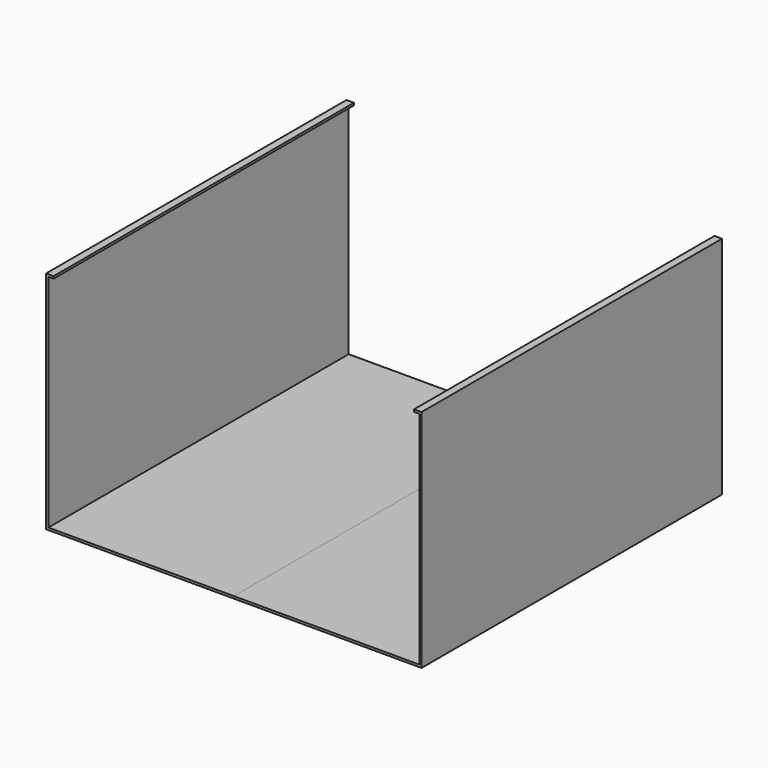
from build123d import *

# Parameters (mm, degrees)
F1_DEPTH = 6350


# Not quite as in the source:
# - a pattern or mirror of a feature is missing from the dataset's text; its kind, count and spacing are read off the source's solid


with BuildPart() as f1:
    # F0 (on Front) → F1 (new body, symmetric)
    with BuildSketch(Plane.XZ):
        Polygon((-6096, 7620), (-6350, 7620), (-6350, 0), (0, 0), (0, 76.2), (-6273.8, 76.2), (-6273.8, 7543.8), (-6096, 7543.8), align=None)
    extrude(amount=F1_DEPTH, both=True)


with BuildPart() as f1_copies_1:
    # F1_copies: instance of F1
    add(f1.part.mirror(Plane(origin=(0, 0, 0), x_dir=(0, 0, 1), z_dir=(1, 0, 0))))


solid = Compound([f1.part, f1_copies_1.part])
